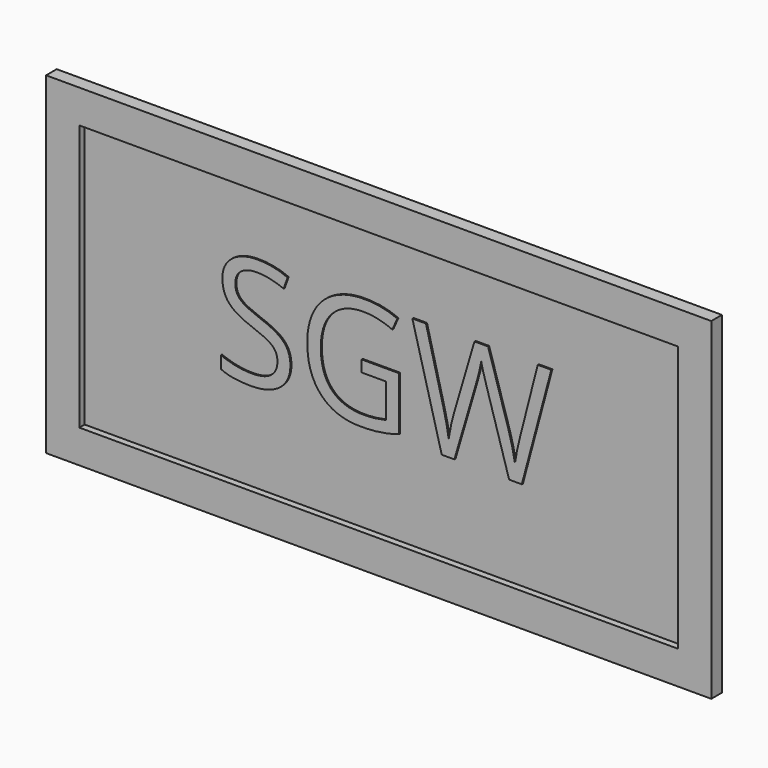
from build123d import *

# Parameters (mm, degrees)
F0_W         = 500
F0_H         = 250
F1_DEPTH     = 10
F2_W         = 450
F2_H         = 200
F3_DEPTH     = 5
F4_W         = 150
F4_H         = 100
F5_DEPTH     = 20
F6_R         = 12.5
F7_DEPTH     = 15
F8_R         = 5
F9_TEXT_SIZE = 116.1902108126
F10_DEPTH    = 1


# Not quite as in the source:
# - Text() gives the source's letters only with a copy of the font that has no kerning and outlines rounded to 1/6400 em; it was checked with that copy


with BuildPart() as f1:
    # F0 (on Front) → F1 (new body)
    with BuildSketch(Plane.XZ):
        with Locations((25.462173009, -18.5891888928)):
            Rectangle(F0_W, F0_H)
    extrude(amount=F1_DEPTH)

    # F2 (on face) → F3 (cut)
    with BuildSketch(Plane.XZ.offset(10)):
        with Locations((25.462173009, -18.5891888928)):
            Rectangle(F2_W, F2_H)
    extrude(amount=-F3_DEPTH, mode=Mode.SUBTRACT)

    # F4 (on face) → F5 (join)
    with BuildSketch(Plane(origin=(0, 0, 0), x_dir=(-1, 0, 0), z_dir=(0, 1, 0))):
        with Locations((-25.462173009, -18.5891888928)):
            Rectangle(F4_W, F4_H)
    extrude(amount=F5_DEPTH)

    # F6 (on face) → F7 (cut)
    with BuildSketch(Plane(origin=(0, 20, 0), x_dir=(-1, 0, 0), z_dir=(0, 1, 0))):
        with Locations((-25.462173009, -18.5891888928)):
            Circle(F6_R)
    extrude(amount=-F7_DEPTH, mode=Mode.SUBTRACT)

    # F8
    f8_edges = [f1.edges().sort_by_distance(p)[0] for p in [
        (100.462173, 10, 31.410811),
        (100.462173, 10, -68.589189),
        (100.462173, 0, -18.589189),
        (100.462173, 20, -18.589189),
        (-49.537827, 10, 31.410811),
        (25.462173, 0, 31.410811),
        (25.462173, 20, 31.410811),
        (-49.537827, 10, -68.589189),
        (-49.537827, 0, -18.589189),
        (-49.537827, 20, -18.589189),
        (25.462173, 0, -68.589189),
        (25.462173, 20, -68.589189),
    ]]
    fillet(f8_edges, radius=F8_R)

    # F9 (on face) → F10 (join)
    with BuildSketch(Plane.XZ.offset(5)):
        with Locations((-102.3107543588, -50.6141148508)):
            Text('SGW', F9_TEXT_SIZE, font='Open Sans', text_align=(TextAlign.LEFT, TextAlign.BOTTOM))
    extrude(amount=F10_DEPTH)


solid = f1.part
